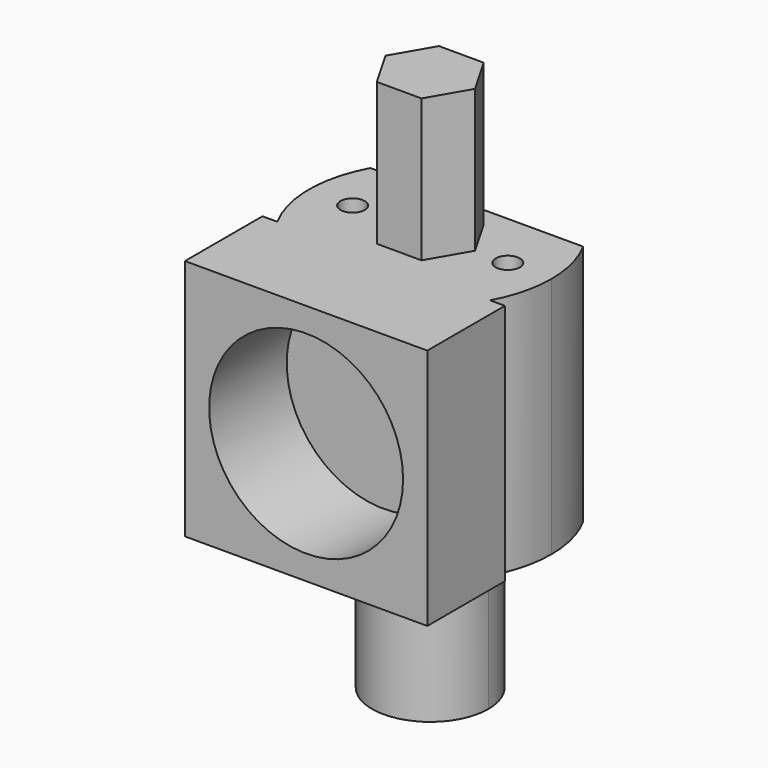
from build123d import *

# Parameters (mm, degrees)
F1_DEPTH  = 25
F3_D      = 2.5
F3_DEPTH  = 13.5
F3_TIP    = 0.7510757738
F4_W      = 21.9317121995
F4_H      = 25
F4_R      = 10
F4_W_2    = 1.5341439003
F5_DEPTH  = 10
F7_DEPTH  = 18.16
F8_SIZE2  = 2
F8_SIZE   = 5.5
F10_DEPTH = 14.7


with BuildPart() as f1:
    # F0 (on Top) → F1 (new body)
    with BuildSketch(Plane.XY):
        with BuildLine():
            ThreePointArc((10.9658560997, -6), (12.1103922572, -3.0965140685), (12.5, 0))
            ThreePointArc((12.5, 0), (12.1103922572, 3.0965140685), (10.9658560997, 6))
            Line((10.9658560997, 6), (-10.9658560997, 6))
            ThreePointArc((-10.9658560997, 6), (-12.5, 0), (-10.9658560997, -6))
            Line((-10.9658560997, -6), (10.9658560997, -6))
        make_face()
    extrude(amount=-F1_DEPTH)

    # F3
    with Locations(Plane.XY):
        with Locations((-8, 0), (8, 0)):
            Hole(F3_D / 2, depth=F3_DEPTH)
            with Locations((0, 0, -(F3_DEPTH + F3_TIP / 2))):  # 118° drill point
                Cone(0, F3_D / 2, F3_TIP, mode=Mode.SUBTRACT)

    # F4 (on face) → F5 (join)
    with BuildSketch(Plane.XZ.offset(6)):
        with Locations((0, -12.5)):
            Rectangle(F4_W, F4_H)
        with Locations((0, -12.5)):
            Circle(F4_R, mode=Mode.SUBTRACT)
        with Locations((-11.7329280499, -12.5)):
            Rectangle(F4_W_2, F4_H)
        with Locations((11.7329280499, -12.5)):
            Rectangle(F4_W_2, F4_H)
    extrude(amount=F5_DEPTH)

    # F6 (on face) → F7 (join)
    with BuildSketch(Plane(origin=(0, 0, -25), x_dir=(1, 0, 0), z_dir=(0, 0, -1))):
        with BuildLine():
            ThreePointArc((0, -6), (4.2426406871, -4.2426406871), (6, 0))
            ThreePointArc((6, 0), (-4.2426406871, 4.2426406871), (0, -6))
        make_face()
    extrude(amount=F7_DEPTH)

    # F8
    f8_edges = [f1.edges().sort_by_distance(p)[0] for p in [
        (0, -6, -43.16),
    ]]
    f8_side = f1.faces().sort_by_distance((0, 0, -43.16))[0]
    chamfer(f8_edges, length=F8_SIZE, length2=F8_SIZE2, reference=f8_side)

    # F9 (on face) → F10 (join)
    with BuildSketch(Plane.XY):
        Polygon((4.6187967668, -0.0070541219), (2.3155074321, 3.996468274), (-2.3032893346, 4.0035223959), (-4.6187967668, 0.0070541219), (-2.3155074321, -3.996468274), (2.3032893346, -4.0035223959), align=None)
    extrude(amount=F10_DEPTH)


solid = f1.part
